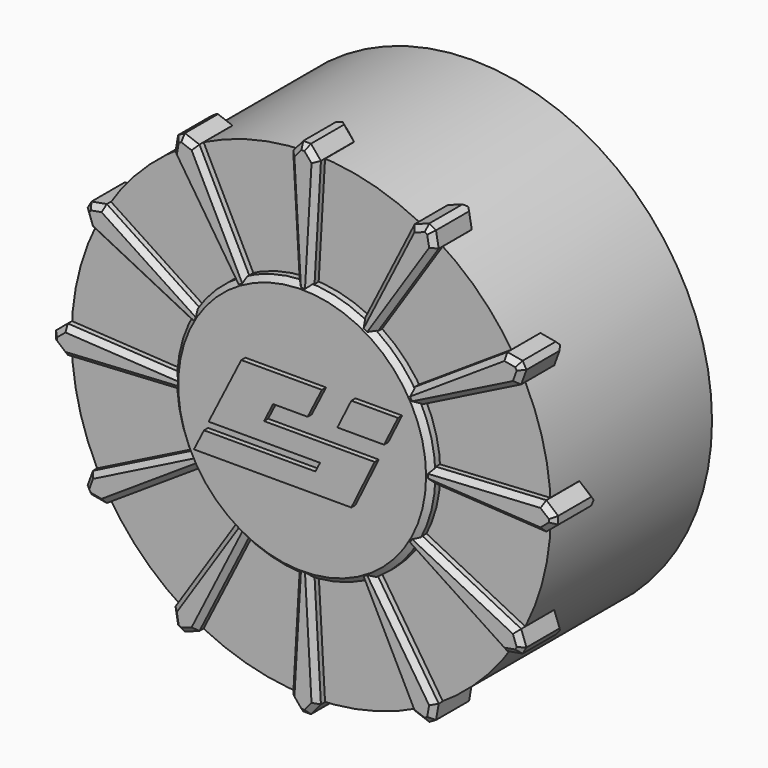
from build123d import *

# Parameters (mm, degrees)
F0_R          = 11.7856
F1_DEPTH      = 9.906
F3_DEPTH      = 8.763
F4_R          = 3.4163
F5_DEPTH      = 2.54
F7_START      = 7.62
F7_DEPTH      = 2.794
F8_C1_SIZE    = 0.508
F8_C2_SIZE    = 0.508
F8_2_C1_SIZE  = 0.508
F8_2_C2_SIZE  = 0.508
F8_3_C1_SIZE  = 0.508
F8_3_C2_SIZE  = 0.508
F8_4_C1_SIZE  = 0.508
F8_4_C2_SIZE  = 0.508
F8_5_C1_SIZE  = 0.508
F8_5_C2_SIZE  = 0.508
F8_6_C1_SIZE  = 0.508
F8_6_C2_SIZE  = 0.508
F8_7_C1_SIZE  = 0.508
F8_7_C2_SIZE  = 0.508
F8_8_C1_SIZE  = 0.508
F8_8_C2_SIZE  = 0.508
F8_9_C1_SIZE  = 0.508
F8_9_C2_SIZE  = 0.508
F8_10_C1_SIZE = 0.508
F8_10_C2_SIZE = 0.508
F8_11_C1_SIZE = 0.508
F8_11_C2_SIZE = 0.508
F8_12_C1_SIZE = 0.508
F8_12_C2_SIZE = 0.508
F9_SIZE2      = 0.254
F9_SIZE       = 0.254
F9_2_SIZE2    = 0.254
F9_2_SIZE     = 0.254
F9_3_SIZE2    = 0.254
F9_3_SIZE     = 0.254
F9_4_SIZE2    = 0.254
F9_4_SIZE     = 0.254
F9_5_SIZE2    = 0.254
F9_5_SIZE     = 0.254
F9_6_SIZE2    = 0.254
F9_6_SIZE     = 0.254
F9_7_SIZE2    = 0.254
F9_7_SIZE     = 0.254
F9_8_SIZE2    = 0.254
F9_8_SIZE     = 0.254
F9_9_SIZE2    = 0.254
F9_9_SIZE     = 0.254
F9_10_SIZE2   = 0.254
F9_10_SIZE    = 0.254
F9_11_SIZE2   = 0.254
F9_11_SIZE    = 0.254
F9_12_SIZE2   = 0.254
F9_12_SIZE    = 0.254
F10_R         = 6.35
F11_DEPTH     = 0.5588
F12_SIZE2     = 0.254
F12_SIZE      = 0.254
F14_DEPTH     = 1.27
F15_SCALE     = 0.28


with BuildPart() as f1:
    # F0 (on Front) → F1 (new body)
    with BuildSketch(Plane.XZ):
        with Locations((-36.2902507186, 18.8595000654)):
            Circle(F0_R)
    extrude(amount=F1_DEPTH)

    # F2 (on face) → F3 (cut)
    with BuildSketch(Plane(origin=(0, 0, 0), x_dir=(-1, 0, 0), z_dir=(0, 1, 0))):
        with BuildLine():
            Line((37.7634507186, 16.2785550835), (37.7634507186, 21.4404450474))
            ThreePointArc((37.7634507186, 21.4404450474), (33.3184507186, 18.8595000654), (37.7634507186, 16.2785550835))
        make_face()
    extrude(amount=-F3_DEPTH, mode=Mode.SUBTRACT)

    # F4 (on face) → F5 (cut)
    with BuildSketch(Plane(origin=(0, 0, 0), x_dir=(-1, 0, 0), z_dir=(0, 1, 0))):
        with Locations((36.2902507186, 18.8595000654)):
            Circle(F4_R)
        with BuildLine():
            Line((37.7634507186, 21.4404450474), (37.7634507186, 16.2785550835))
            ThreePointArc((37.7634507186, 16.2785550835), (33.3184507186, 18.8595000654), (37.7634507186, 21.4404450474))
        make_face(mode=Mode.SUBTRACT)
    extrude(amount=-F5_DEPTH, mode=Mode.SUBTRACT)


with BuildPart() as f7:
    # F6 (on Front) → F7 (new body)
    with BuildSketch(Plane.XZ.offset(F7_START)):
        Polygon((-25.7604879888, 13.5656862971), (-36.2902507186, 18.8595000654), (-26.4407921474, 12.3873649298), (-25.6903686396, 12.5196848412), (-25.4998686396, 12.84964052), align=None)
    extrude(amount=F7_DEPTH)

    # F8: chamfer of 0.508 on 3 edges, made by hand

    # F8_c1
    f8_c1_edges = [f7.edges().sort_by_distance(p)[0] for p in [
        (-25.6301783142, -7.62, 13.2076634086),
    ]]
    chamfer(f8_c1_edges, length=F8_C1_SIZE)

    # F8_c2
    f8_c2_edges = [f7.edges().sort_by_distance(p)[0] for p in [
        (-26.1736489271, -7.62, 12.4344694873),
    ]]
    chamfer(f8_c2_edges, length=F8_C2_SIZE)

    # F9
    f9_edges = [f7.edges().sort_by_distance(p)[0] for p in [
        (-25.595119, -10.414, 12.684663),
        (-25.630178, -10.414, 13.207663),
        (-31.025369, -10.414, 16.212593),
        (-31.365521, -10.414, 15.623432),
        (-26.06558, -10.414, 12.453525),
    ]]
    chamfer(f9_edges, length=F9_SIZE, length2=F9_SIZE2)


with BuildPart() as f7b:
    # F6 (on Front) → F7, piece 2 (new body)
    with BuildSketch(Plane.XZ.offset(F7_START)):
        Polygon((-24.5243018146, 19.539804224), (-36.2902507186, 18.8595000654), (-24.5243018146, 18.1791959069), (-23.9405759489, 18.6690000654), (-23.9405759489, 19.0500000654), align=None)
    extrude(amount=F7_DEPTH)

    # F8#2: chamfer of 0.508 on 3 edges, made by hand

    # F8_2_c1
    f8_2_c1_edges = [f7b.edges().sort_by_distance(p)[0] for p in [
        (-24.2324388818, -7.62, 19.2949021447),
    ]]
    chamfer(f8_2_c1_edges, length=F8_2_C1_SIZE)

    # F8_2_c2
    f8_2_c2_edges = [f7b.edges().sort_by_distance(p)[0] for p in [
        (-24.3165012781, -7.62, 18.3535612604),
    ]]
    chamfer(f8_2_c2_edges, length=F8_2_C2_SIZE)

    # F9#2
    f9_2_edges = [f7b.edges().sort_by_distance(p)[0] for p in [
        (-23.940576, -10.414, 18.8595),
        (-24.232439, -10.414, 19.294902),
        (-30.407276, -10.414, 19.199652),
        (-30.407276, -10.414, 18.519348),
        (-24.232439, -10.414, 18.424098),
    ]]
    chamfer(f9_2_edges, length=F9_2_SIZE, length2=F9_2_SIZE2)


with BuildPart() as f7c:
    # F6 (on Front) → F7, piece 3 (new body)
    with BuildSketch(Plane.XZ.offset(F7_START)):
        Polygon((-26.4407921474, 25.3316352011), (-36.2902507186, 18.8595000654), (-25.7604879888, 24.1533138338), (-25.4998686396, 24.8693596109), (-25.6903686396, 25.1993152897), align=None)
    extrude(amount=F7_DEPTH)

    # F8#3: chamfer of 0.508 on 3 edges, made by hand

    # F8_3_c1
    f8_3_c1_edges = [f7c.edges().sort_by_distance(p)[0] for p in [
        (-26.0655803935, -7.62, 25.2654752454),
    ]]
    chamfer(f8_3_c1_edges, length=F8_3_C1_SIZE)

    # F8_3_c2
    f8_3_c2_edges = [f7c.edges().sort_by_distance(p)[0] for p in [
        (-25.667710122, -7.62, 24.4082189278),
    ]]
    chamfer(f8_3_c2_edges, length=F8_3_C2_SIZE)

    # F9#3
    f9_3_edges = [f7c.edges().sort_by_distance(p)[0] for p in [
        (-25.595119, -10.414, 25.034337),
        (-26.06558, -10.414, 25.265475),
        (-31.365521, -10.414, 22.095568),
        (-31.025369, -10.414, 21.506407),
        (-25.630178, -10.414, 24.511337),
    ]]
    chamfer(f9_3_edges, length=F9_3_SIZE, length2=F9_3_SIZE2)


with BuildPart() as f7d:
    # F6 (on Front) → F7, piece 4 (new body)
    with BuildSketch(Plane.XZ.offset(F7_START)):
        Polygon((-30.9964369502, 29.3892627952), (-36.2902507186, 18.8595000654), (-29.818115583, 28.7089586367), (-29.9504354943, 29.4593821445), (-30.2803911732, 29.6498821445), align=None)
    extrude(amount=F7_DEPTH)

    # F8#4: chamfer of 0.508 on 3 edges, made by hand

    # F8_4_c1
    f8_4_c1_edges = [f7d.edges().sort_by_distance(p)[0] for p in [
        (-29.8842755386, -7.62, 29.0841703906),
    ]]
    chamfer(f8_4_c1_edges, length=F8_4_C1_SIZE)

    # F8_4_c2
    f8_4_c2_edges = [f7d.edges().sort_by_distance(p)[0] for p in [
        (-30.7415318563, -7.62, 29.482040662),
    ]]
    chamfer(f8_4_c2_edges, length=F8_4_C2_SIZE)

    # F9#4
    f9_4_edges = [f7d.edges().sort_by_distance(p)[0] for p in [
        (-30.115413, -10.414, 29.554632),
        (-30.638414, -10.414, 29.519572),
        (-33.643344, -10.414, 24.124381),
        (-33.054183, -10.414, 23.784229),
        (-29.884276, -10.414, 29.08417),
    ]]
    chamfer(f9_4_edges, length=F9_4_SIZE, length2=F9_4_SIZE2)


with BuildPart() as f7e:
    # F6 (on Front) → F7, piece 5 (new body)
    with BuildSketch(Plane.XZ.offset(F7_START)):
        Polygon((-36.4807507186, 31.2091748351), (-36.9705548772, 30.6254489695), (-36.2902507186, 18.8595000654), (-35.60994656, 30.6254489695), (-36.0997507186, 31.2091748351), align=None)
    extrude(amount=F7_DEPTH)

    # F8#5: chamfer of 0.508 on 3 edges, made by hand

    # F8_5_c1
    f8_5_c1_edges = [f7e.edges().sort_by_distance(p)[0] for p in [
        (-36.7256527979, -7.62, 30.9173119023),
    ]]
    chamfer(f8_5_c1_edges, length=F8_5_C1_SIZE)

    # F8_5_c2
    f8_5_c2_edges = [f7e.edges().sort_by_distance(p)[0] for p in [
        (-35.7843119136, -7.62, 30.833249506),
    ]]
    chamfer(f8_5_c2_edges, length=F8_5_C2_SIZE)

    # F9#5
    f9_5_edges = [f7e.edges().sort_by_distance(p)[0] for p in [
        (-36.725653, -10.414, 30.917312),
        (-36.630403, -10.414, 24.742475),
        (-35.950099, -10.414, 24.742475),
        (-35.854849, -10.414, 30.917312),
        (-36.290251, -10.414, 31.209175),
    ]]
    chamfer(f9_5_edges, length=F9_5_SIZE, length2=F9_5_SIZE2)


with BuildPart() as f7f:
    # F6 (on Front) → F7, piece 6 (new body)
    with BuildSketch(Plane.XZ.offset(F7_START)):
        Polygon((-46.8200134484, 24.1533138338), (-36.2902507186, 18.8595000654), (-46.1397092898, 25.3316352011), (-46.8901327976, 25.1993152897), (-47.0806327976, 24.8693596109), align=None)
    extrude(amount=F7_DEPTH)

    # F8#6: chamfer of 0.508 on 3 edges, made by hand

    # F8_6_c1
    f8_6_c1_edges = [f7f.edges().sort_by_distance(p)[0] for p in [
        (-46.950323123, -7.62, 24.5113367223),
    ]]
    chamfer(f8_6_c1_edges, length=F8_6_C1_SIZE)

    # F8_6_c2
    f8_6_c2_edges = [f7f.edges().sort_by_distance(p)[0] for p in [
        (-46.4068525101, -7.62, 25.2845306436),
    ]]
    chamfer(f8_6_c2_edges, length=F8_6_C2_SIZE)

    # F9#6
    f9_6_edges = [f7f.edges().sort_by_distance(p)[0] for p in [
        (-46.985383, -10.414, 25.034337),
        (-46.950323, -10.414, 24.511337),
        (-41.555132, -10.414, 21.506407),
        (-41.21498, -10.414, 22.095568),
        (-46.514921, -10.414, 25.265475),
    ]]
    chamfer(f9_6_edges, length=F9_6_SIZE, length2=F9_6_SIZE2)


with BuildPart() as f7g:
    # F6 (on Front) → F7, piece 7 (new body)
    with BuildSketch(Plane.XZ.offset(F7_START)):
        Polygon((-48.0561996226, 18.1791959069), (-36.2902507186, 18.8595000654), (-48.0561996226, 19.539804224), (-48.6399254883, 19.0500000654), (-48.6399254883, 18.6690000654), align=None)
    extrude(amount=F7_DEPTH)

    # F8#7: chamfer of 0.508 on 3 edges, made by hand

    # F8_7_c1
    f8_7_c1_edges = [f7g.edges().sort_by_distance(p)[0] for p in [
        (-48.3480625554, -7.62, 18.4240979862),
    ]]
    chamfer(f8_7_c1_edges, length=F8_7_C1_SIZE)

    # F8_7_c2
    f8_7_c2_edges = [f7g.edges().sort_by_distance(p)[0] for p in [
        (-48.2640001591, -7.62, 19.3654388705),
    ]]
    chamfer(f8_7_c2_edges, length=F8_7_C2_SIZE)

    # F9#7
    f9_7_edges = [f7g.edges().sort_by_distance(p)[0] for p in [
        (-48.348063, -10.414, 18.424098),
        (-42.173225, -10.414, 18.519348),
        (-42.173225, -10.414, 19.199652),
        (-48.348063, -10.414, 19.294902),
        (-48.639925, -10.414, 18.8595),
    ]]
    chamfer(f9_7_edges, length=F9_7_SIZE, length2=F9_7_SIZE2)


with BuildPart() as f7h:
    # F6 (on Front) → F7, piece 8 (new body)
    with BuildSketch(Plane.XZ.offset(F7_START)):
        Polygon((-46.1397092898, 12.3873649298), (-36.2902507186, 18.8595000654), (-46.8200134484, 13.5656862971), (-47.0806327976, 12.84964052), (-46.8901327976, 12.5196848412), align=None)
    extrude(amount=F7_DEPTH)

    # F8#8: chamfer of 0.508 on 3 edges, made by hand

    # F8_8_c1
    f8_8_c1_edges = [f7h.edges().sort_by_distance(p)[0] for p in [
        (-46.5149210437, -7.62, 12.4535248855),
    ]]
    chamfer(f8_8_c1_edges, length=F8_8_C1_SIZE)

    # F8_8_c2
    f8_8_c2_edges = [f7h.edges().sort_by_distance(p)[0] for p in [
        (-46.9127913152, -7.62, 13.3107812031),
    ]]
    chamfer(f8_8_c2_edges, length=F8_8_C2_SIZE)

    # F9#8
    f9_8_edges = [f7h.edges().sort_by_distance(p)[0] for p in [
        (-46.514921, -10.414, 12.453525),
        (-41.21498, -10.414, 15.623432),
        (-41.555132, -10.414, 16.212593),
        (-46.950323, -10.414, 13.207663),
        (-46.985383, -10.414, 12.684663),
    ]]
    chamfer(f9_8_edges, length=F9_8_SIZE, length2=F9_8_SIZE2)


with BuildPart() as f7i:
    # F6 (on Front) → F7, piece 9 (new body)
    with BuildSketch(Plane.XZ.offset(F7_START)):
        Polygon((-41.584064487, 8.3297373357), (-36.2902507186, 18.8595000654), (-42.7623858542, 9.0100414942), (-42.6300659428, 8.2596179864), (-42.300110264, 8.0691179864), align=None)
    extrude(amount=F7_DEPTH)

    # F8#9: chamfer of 0.508 on 3 edges, made by hand

    # F8_9_c1
    f8_9_c1_edges = [f7i.edges().sort_by_distance(p)[0] for p in [
        (-41.9420873755, -7.62, 8.199427661),
    ]]
    chamfer(f8_9_c1_edges, length=F8_9_C1_SIZE)

    # F8_9_c2
    f8_9_c2_edges = [f7i.edges().sort_by_distance(p)[0] for p in [
        (-42.7152812968, -7.62, 8.7428982739),
    ]]
    chamfer(f8_9_c2_edges, length=F8_9_C2_SIZE)

    # F9#9
    f9_9_edges = [f7i.edges().sort_by_distance(p)[0] for p in [
        (-42.465088, -10.414, 8.164368),
        (-41.942087, -10.414, 8.199428),
        (-38.937158, -10.414, 13.594619),
        (-39.526318, -10.414, 13.934771),
        (-42.696226, -10.414, 8.63483),
    ]]
    chamfer(f9_9_edges, length=F9_9_SIZE, length2=F9_9_SIZE2)


with BuildPart() as f7j:
    # F6 (on Front) → F7, piece 10 (new body)
    with BuildSketch(Plane.XZ.offset(F7_START)):
        Polygon((-35.60994656, 7.0935511614), (-36.2902507186, 18.8595000654), (-36.9705548772, 7.0935511614), (-36.4807507186, 6.5098252958), (-36.0997507186, 6.5098252958), align=None)
    extrude(amount=F7_DEPTH)

    # F8#10: chamfer of 0.508 on 3 edges, made by hand

    # F8_10_c1
    f8_10_c1_edges = [f7j.edges().sort_by_distance(p)[0] for p in [
        (-35.8548486393, -7.62, 6.8016882286),
    ]]
    chamfer(f8_10_c1_edges, length=F8_10_C1_SIZE)

    # F8_10_c2
    f8_10_c2_edges = [f7j.edges().sort_by_distance(p)[0] for p in [
        (-36.7961895236, -7.62, 6.8857506249),
    ]]
    chamfer(f8_10_c2_edges, length=F8_10_C2_SIZE)

    # F9#10
    f9_10_edges = [f7j.edges().sort_by_distance(p)[0] for p in [
        (-36.290251, -10.414, 6.509825),
        (-35.854849, -10.414, 6.801688),
        (-35.950099, -10.414, 12.976526),
        (-36.630403, -10.414, 12.976526),
        (-36.725653, -10.414, 6.801688),
    ]]
    chamfer(f9_10_edges, length=F9_10_SIZE, length2=F9_10_SIZE2)


with BuildPart() as f7k:
    # F6 (on Front) → F7, piece 11 (new body)
    with BuildSketch(Plane.XZ.offset(F7_START)):
        Polygon((-29.818115583, 9.0100414942), (-36.2902507186, 18.8595000654), (-30.9964369502, 8.3297373357), (-30.2803911732, 8.0691179864), (-29.9504354943, 8.2596179864), align=None)
    extrude(amount=F7_DEPTH)

    # F8#11: chamfer of 0.508 on 3 edges, made by hand

    # F8_11_c1
    f8_11_c1_edges = [f7k.edges().sort_by_distance(p)[0] for p in [
        (-29.8842755386, -7.62, 8.6348297403),
    ]]
    chamfer(f8_11_c1_edges, length=F8_11_C1_SIZE)

    # F8_11_c2
    f8_11_c2_edges = [f7k.edges().sort_by_distance(p)[0] for p in [
        (-30.7415318563, -7.62, 8.2369594689),
    ]]
    chamfer(f8_11_c2_edges, length=F8_11_C2_SIZE)

    # F9#11
    f9_11_edges = [f7k.edges().sort_by_distance(p)[0] for p in [
        (-30.115413, -10.414, 8.164368),
        (-29.884276, -10.414, 8.63483),
        (-33.054183, -10.414, 13.934771),
        (-33.643344, -10.414, 13.594619),
        (-30.638414, -10.414, 8.199428),
    ]]
    chamfer(f9_11_edges, length=F9_11_SIZE, length2=F9_11_SIZE2)


with BuildPart() as f7l:
    # F6 (on Front) → F7, piece 12 (new body)
    with BuildSketch(Plane.XZ.offset(F7_START)):
        Polygon((-42.7623858542, 28.7089586367), (-36.2902507186, 18.8595000654), (-41.584064487, 29.3892627952), (-42.300110264, 29.6498821445), (-42.6300659428, 29.4593821445), align=None)
    extrude(amount=F7_DEPTH)

    # F8#12: chamfer of 0.508 on 3 edges, made by hand

    # F8_12_c1
    f8_12_c1_edges = [f7l.edges().sort_by_distance(p)[0] for p in [
        (-42.6962258985, -7.62, 29.0841703906),
    ]]
    chamfer(f8_12_c1_edges, length=F8_12_C1_SIZE)

    # F8_12_c2
    f8_12_c2_edges = [f7l.edges().sort_by_distance(p)[0] for p in [
        (-41.8389695809, -7.62, 29.482040662),
    ]]
    chamfer(f8_12_c2_edges, length=F8_12_C2_SIZE)

    # F9#12
    f9_12_edges = [f7l.edges().sort_by_distance(p)[0] for p in [
        (-42.696226, -10.414, 29.08417),
        (-39.526318, -10.414, 23.784229),
        (-38.937158, -10.414, 24.124381),
        (-41.942087, -10.414, 29.519572),
        (-42.465088, -10.414, 29.554632),
    ]]
    chamfer(f9_12_edges, length=F9_12_SIZE, length2=F9_12_SIZE2)


with BuildPart() as f11:
    # F10 (on face) → F11 (new body)
    with BuildSketch(Plane.XZ.offset(9.906)):
        with Locations((-36.2902507186, 18.8595000654)):
            Circle(F10_R)
    extrude(amount=F11_DEPTH)

    # F12
    f12_edges = [f11.edges().sort_by_distance(p)[0] for p in [
        (-42.640251, -10.4648, 18.8595),
    ]]
    chamfer(f12_edges, length=F12_SIZE, length2=F12_SIZE2)


with BuildPart() as f14:
    # F13 (on face) → F14 (new body)
    with BuildSketch(Plane.XZ.offset(10.4648)):
        Polygon((16.3267976039, 7.5823681484), (8.1284711503, 7.5823681484), (5.6759848936, 2.6415927166), (13.8743113471, 2.6415927166), align=None)
    extrude(amount=F14_DEPTH)


with BuildPart() as f14b:
    # F13 (on face) → F14, piece 2 (new body)
    with BuildSketch(Plane.XZ.offset(10.4648)):
        Polygon((2.966908565, 7.5823681484), (-11.2004294626, 7.5823681484), (-16.9379295517, -3.8100776187), (2.6306693929, -3.8100776187), (1.8358969263, -5.4112251342), (-17.7443046006, -5.4112251342), (-19.5184401802, -8.9339690228), (8.1284711503, -8.9339690228), (12.2276343771, -0.5574927701), (-7.2009206262, -0.5574927701), (-5.6127803966, 2.5959366253), (0.4556259228, 2.5959366253), align=None)
    extrude(amount=F14_DEPTH)


with BuildPart() as f14b_1:
    # F15: moved
    add(f14b.part.scale(F15_SCALE).moved(Location((-5.1846628509, -8.449056, -0.4013947945))))


with BuildPart() as f14_1:
    # F15: moved
    add(f14.part.scale(F15_SCALE).moved(Location((-5.1846628509, -8.449056, -0.4013947945))))


with BuildPart() as f14b_2:
    # F16: moved
    add(f14b_1.part.moved(Location((-30.7594, 0, 19.3802))))


with BuildPart() as f14_2:
    # F16: moved
    add(f14_1.part.moved(Location((-30.7594, 0, 19.3802))))


with BuildPart() as f14b_3:
    # F17: moved
    add(f14b_2.part.moved(Location((0, 1.016, 0))))


with BuildPart() as f14_3:
    # F17: moved
    add(f14_2.part.moved(Location((0, 1.016, 0))))


solid = Compound([f1.part, f7.part, f7b.part, f7c.part, f7d.part, f7e.part, f7f.part, f7g.part, f7h.part, f7i.part, f7j.part, f7k.part, f7l.part, f11.part, f14b_3.part, f14_3.part])
